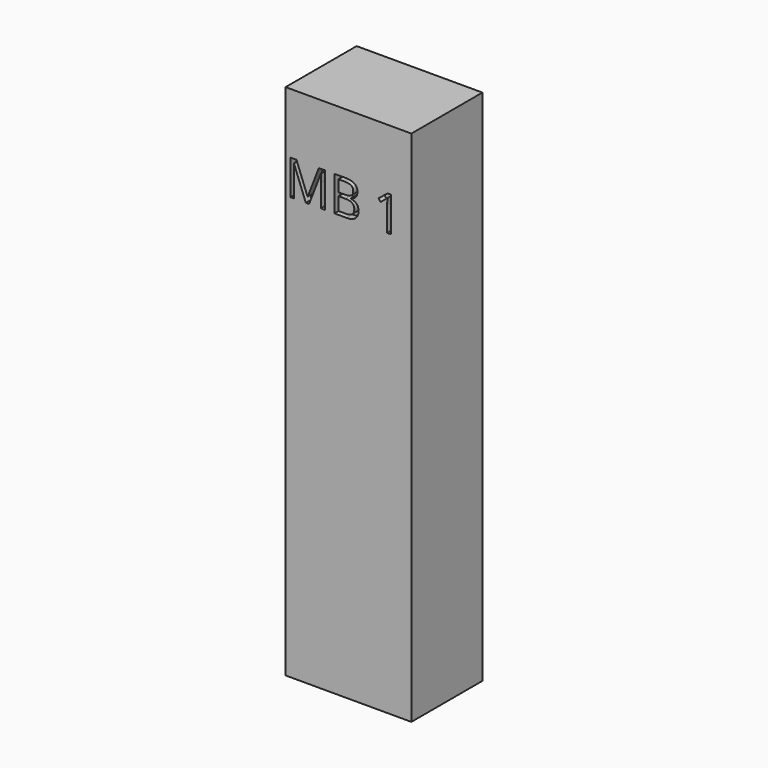
from build123d import *

# Parameters (mm, degrees)
F0_W         = 431.8
F0_H         = 1778
F1_DEPTH     = 152.4
F2_TEXT_SIZE = 167.5892620232
F3_DEPTH     = 25.4


# Not quite as in the source:
# - Text() gives the source's letters only with a copy of the font that has no kerning and outlines rounded to 1/6400 em; it was checked with that copy


with BuildPart() as f1:
    # F0 (on Front) → F1 (new body, symmetric)
    with BuildSketch(Plane.XZ):
        Rectangle(F0_W, F0_H)
    extrude(amount=F1_DEPTH, both=True)

    # F2 (on face) → F3 (cut)
    with BuildSketch(Plane.XZ.offset(152.4)):
        with Locations((-215.9, 561.8143081665)):
            Text('MB 1', F2_TEXT_SIZE, font='Open Sans', text_align=(TextAlign.LEFT, TextAlign.BOTTOM))
    extrude(amount=-F3_DEPTH, mode=Mode.SUBTRACT)


solid = f1.part
